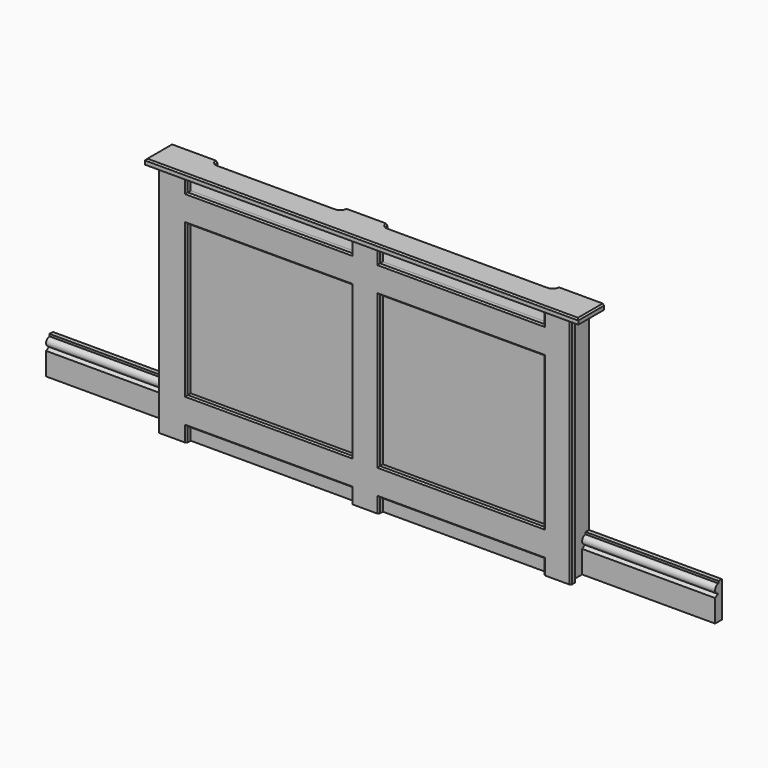
from build123d import *

# Parameters (mm, degrees)
F0_W          = 1340
F0_H          = 80
F1_DEPTH      = 770
F3_DEPTH      = 500
F3_DEPTH_BACK = 1840
F4_W          = 15
F4_H          = 820
F4_W_2        = 576
F4_H_2        = 528
F4_W_3        = 96
F4_H_3        = 50
F4_W_4        = 18
F5_DEPTH      = 18
F6_SIZE       = 5
F7_DEPTH      = 63
F7_DEPTH_BACK = 33
F8_SIZE       = 5
F9_DEPTH      = 80
F11_DEPTH     = 18
F12_SIZE      = 4.99999


# Not quite as in the source:
# - a fillet or chamfer is up to 0.001 mm smaller than in the source, because OpenCascade refuses the exact size


with BuildPart() as f1:
    # F0 (on Top) → F1 (new body)
    with BuildSketch(Plane.XY):
        with Locations((609.8307800293, -4.9345558882)):
            Rectangle(F0_W, F0_H)
    extrude(amount=F1_DEPTH)

    # F2 (on face) → F3 (join, two sides)
    with BuildSketch(Plane(origin=(-60.1692199707, 0, 0), x_dir=(0, -1, 0), z_dir=(-1, 0, 0))) as f3_sk:
        with BuildLine():
            Line((-35.0654441118, 125), (-35.0654441118, 0))
            Line((-35.0654441118, 0), (-5.2516935417, 0))
            Line((-5.2516935417, 0), (-5.2516935417, 78.7325807151))
            Line((-5.2516935417, 78.7325807151), (-20.2490844093, 87.3992991551))
            ThreePointArc((-20.2490844093, 87.3992991551), (-5.2490844093, 102.3992991551), (-20.2490844093, 117.3992991551))
            Line((-20.2490844093, 117.3992991551), (-20.2490844093, 125))
            Line((-20.2490844093, 125), (-35.0654441118, 125))
        make_face()
    extrude(amount=F3_DEPTH)
    extrude(f3_sk.sketch, amount=-F3_DEPTH_BACK)


with BuildPart() as f5:
    # F4 (on face) → F5 (new body)
    with BuildSketch(Plane.XZ.offset(44.9345558882)):
        with Locations((-102.6692199707, 410)):
            Rectangle(F4_W, F4_H)
        Polygon((657.8307800293, 770), (561.8307800293, 770), (-14.1692199707, 770), (-60.1692199707, 770), (-60.1692199707, 0), (-14.1692199707, 0), (-14.1692199707, 50), (561.8307800293, 50), (561.8307800293, 0), (657.8307800293, 0), (657.8307800293, 50), (1233.8307800293, 50), (1233.8307800293, 0), (1279.8307800293, 0), (1279.8307800293, 770), (1233.8307800293, 770), align=None)
        with Locations((273.8307800293, 410)):
            Rectangle(F4_W_2, F4_H_2, mode=Mode.SUBTRACT)
        with Locations((945.8307800293, 410)):
            Rectangle(F4_W_2, F4_H_2, mode=Mode.SUBTRACT)
        with Locations((609.8307800293, 795)):
            Rectangle(F4_W_3, F4_H_3)
        with Locations((1322.3307800293, 410)):
            Rectangle(F4_W, F4_H)
        Polygon((-14.1692199707, 770), (-14.1692199707, 820), (-77.1692199707, 820), (-77.1692199707, 0), (-60.1692199707, 0), (-60.1692199707, 770), align=None)
        with Locations((-86.1692199707, 410)):
            Rectangle(F4_W_4, F4_H)
        Polygon((1296.8307800293, 820), (1233.8307800293, 820), (1233.8307800293, 770), (1279.8307800293, 770), (1279.8307800293, 0), (1296.8307800293, 0), align=None)
        with Locations((1305.8307800293, 410)):
            Rectangle(F4_W_4, F4_H)
    extrude(amount=F5_DEPTH)

    # F6
    f6_edges = [f5.edges().sort_by_distance(p)[0] for p in [
        (-14.16922, -62.934556, 795),
        (273.83078, -62.934556, 770),
        (561.83078, -62.934556, 795),
        (657.83078, -62.934556, 795),
        (945.83078, -62.934556, 770),
        (1233.83078, -62.934556, 795),
        (1233.83078, -62.934556, 410),
        (945.83078, -62.934556, 674),
        (657.83078, -62.934556, 410),
        (945.83078, -62.934556, 146),
        (561.83078, -62.934556, 410),
        (273.83078, -62.934556, 674),
        (-14.16922, -62.934556, 410),
        (273.83078, -62.934556, 146),
        (-14.16922, -62.934556, 25),
        (273.83078, -62.934556, 50),
        (561.83078, -62.934556, 25),
        (657.83078, -62.934556, 25),
        (945.83078, -62.934556, 50),
        (1233.83078, -62.934556, 25),
        (1329.83078, -62.934556, 410),
    ]]
    chamfer(f6_edges, length=F6_SIZE)


with BuildPart() as f7:
    # F4 (on face) → F7 (new body, two sides)
    with BuildSketch(Plane.XZ.offset(44.9345558882)) as f7_sk:
        Polygon((-14.1692199707, 820), (561.8307800293, 820), (657.8307800293, 820), (1233.8307800293, 820), (1296.8307800293, 820), (1314.8307800293, 820), (1329.8307800293, 820), (1367.8307800293, 820), (1367.8307800293, 838), (-148.1692199707, 838), (-148.1692199707, 820), (-110.1692199707, 820), (-95.1692199707, 820), (-77.1692199707, 820), align=None)
    extrude(amount=-F7_DEPTH)
    extrude(f7_sk.sketch, amount=F7_DEPTH_BACK)

    # F8
    f8_edges = [f7.edges().sort_by_distance(p)[0] for p in [
        (-148.16922, -29.934556, 838),
        (609.83078, -77.934556, 838),
        (1367.83078, -29.934556, 838),
    ]]
    chamfer(f8_edges, length=F8_SIZE)

    # F10 (on face) → F11 (join)
    with BuildSketch(Plane.XY.offset(838)):
        with BuildLine():
            Line((-60.1692199707, 35.0654441118), (-148.1692199707, 35.0654441118))
            Line((-148.1692199707, 35.0654441118), (-148.1692199707, 18.0654441118))
            Line((-148.1692199707, 18.0654441118), (-143.1692199707, 18.0654441118))
            Line((-143.1692199707, 18.0654441118), (31.8307800574, 18.0654441118))
            ThreePointArc((31.8307800574, 18.0654441118), (19.8099647591, 23.0446288217), (14.8307800293, 35.0654441118))
            Line((14.8307800293, 35.0654441118), (-60.1692199707, 35.0654441118))
        make_face()
        with BuildLine():
            ThreePointArc((461.8307800293, 35.0654441118), (456.8515952122, 23.0446287344), (444.8307797541, 18.0654441118))
            Line((444.8307797541, 18.0654441118), (626.8307800293, 18.0654441118))
            ThreePointArc((626.8307800293, 18.0654441118), (614.8099647491, 23.0446288317), (609.8307800293, 35.0654441118))
            Line((609.8307800293, 35.0654441118), (461.8307800293, 35.0654441118))
        make_face()
        with BuildLine():
            Line((1187.8307800293, 18.0654441118), (1362.8307800293, 18.0654441118))
            Line((1362.8307800293, 18.0654441118), (1367.8307800293, 18.0654441118))
            Line((1367.8307800293, 18.0654441118), (1367.8307800293, 35.0654441118))
            Line((1367.8307800293, 35.0654441118), (1279.8307800293, 35.0654441118))
            Line((1279.8307800293, 35.0654441118), (1204.8307800293, 35.0654441118))
            ThreePointArc((1204.8307800293, 35.0654441118), (1199.8515953095, 23.0446288317), (1187.8307800293, 18.0654441118))
        make_face()
    extrude(amount=-F11_DEPTH)

    # F12 (size 5 in the source; OpenCascade refuses exactly that, so slightly less here)
    f12_edges = [f7.edges().sort_by_distance(p)[0] for p in [
        (1367.83078, 26.565444, 838),
        (1199.851595, 23.044629, 838),
        (456.851595, 23.044629, 838),
        (-148.16922, 26.565444, 838),
    ]]
    chamfer(f12_edges, length=F12_SIZE)


with BuildPart() as f9:
    # F4 (on face) → F9 (new body)
    with BuildSketch(Plane.XZ.offset(44.9345558882)):
        with Locations((-86.1692199707, 410)):
            Rectangle(F4_W_4, F4_H)
    extrude(amount=-F9_DEPTH)


with BuildPart() as f9b:
    # F4 (on face) → F9, piece 2 (new body)
    with BuildSketch(Plane.XZ.offset(44.9345558882)):
        with Locations((1305.8307800293, 410)):
            Rectangle(F4_W_4, F4_H)
    extrude(amount=-F9_DEPTH)


solid = Compound([f1.part, f5.part, f7.part, f9.part, f9b.part])
